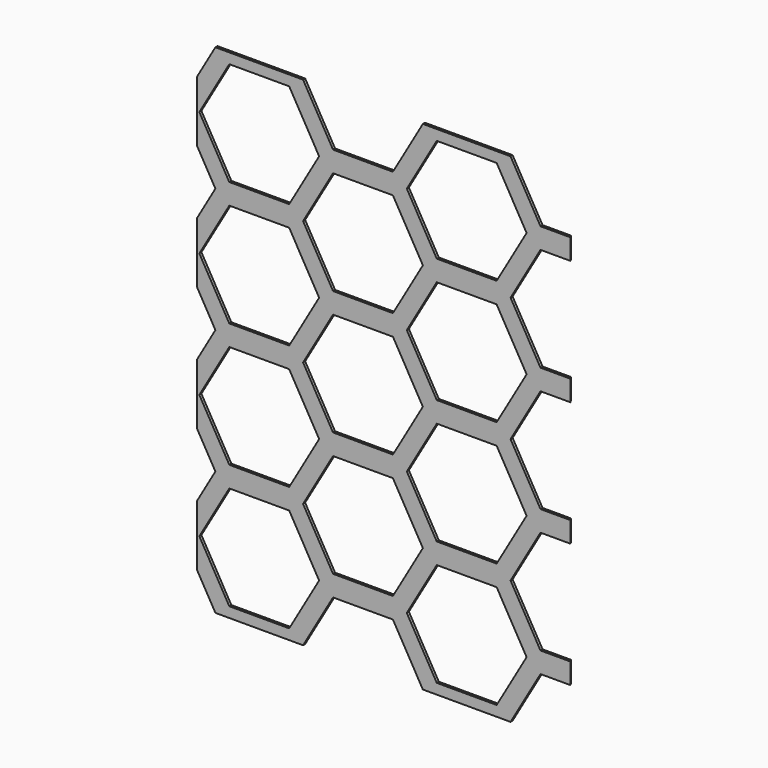
from build123d import *

# Parameters (mm, degrees)
F1_DEPTH    = 3.175
F2_T1_DEPTH = 41.9033921872
F3_T1_DEPTH = 42.5180012054
F4_T1_DEPTH = 41.9033921872
F5_T1_DEPTH = 41.9033921872


# Not quite as in the source:
# - a fillet or chamfer that OpenCascade refuses, or shapes differently, is made with other operations: its cross-section is extruded or revolved along the edge and cut away or added
# - ends of sketch curves that miss each other by under 0.0002 mm in the source are joined


with BuildPart() as f1:
    # F0 (on Front) → F1 (new body)
    with BuildSketch(Plane.XZ):
        Polygon((-134.9552678654, 118.4551059571), (-242.3083075974, 118.4551059571), (-264.8317917845, 79.4432945156), (-264.8317917845, 5.0669305831), (-242.3083075974, -33.9448883924), (-264.8317917845, -72.9567073679), (-264.8317917845, -147.3330713004), (-242.3083075974, -186.3448902759), (-264.8317917845, -225.3567092514), (-264.8317917845, -299.7330731839), (-242.3083075974, -338.7448921594), (-264.8317917845, -377.7567111349), (-264.8317917845, -452.1330750674), (-242.3083075974, -491.1448940429), (-134.9552678654, -491.1448940429), (-98.2935257718, -427.6448940429), (-24.9700415847, -427.6448940429), (11.6917005088, -491.1448940429), (119.0447402409, -491.1448940429), (155.7064823344, -427.6448940429), (192.3682082155, -427.6448940429), (192.3682082155, -402.2448921594), (155.7064823344, -402.2448921594), (119.0447402409, -338.7448921594), (155.7064823344, -275.2448921594), (192.3682082155, -275.2448921594), (192.3682082155, -249.8448902759), (155.7064823344, -249.8448902759), (119.0447402409, -186.3448902759), (155.7064823344, -122.8448902759), (192.3682082155, -122.8448902759), (192.3682082155, -97.4448883924), (155.7064823344, -97.4448883924), (119.0447402409, -33.9448883924), (155.7064823344, 29.5551116076), (192.3682082155, 29.5551116076), (192.3682082155, 54.9551134911), (155.7064823344, 54.9551134911), (119.0447402409, 118.4551134911), (11.6917005088, 118.4551059571), (-24.9700415847, 54.9551134911), (-98.2935257718, 54.9551134911), align=None)
        Polygon((-261.9552759716, -414.9448940429), (-225.2935338781, -351.4448940429), (-151.970049691, -351.4448940429), (-115.3083075974, -414.9448940429), (-151.970049691, -478.4448940429), (-225.2935338781, -478.4448940429), align=None, mode=Mode.SUBTRACT)
        Polygon((11.6917005088, -338.7448921594), (-24.9700415847, -402.2448921594), (-98.2935257718, -402.2448921594), (-134.9552678654, -338.7448921594), (-98.2935257718, -275.2448921594), (-24.9700415847, -275.2448921594), align=None, mode=Mode.SUBTRACT)
        Polygon((-115.3083075974, -262.5448921594), (-151.970049691, -326.0448921594), (-225.2935338781, -326.0448921594), (-261.9552759716, -262.5448921594), (-225.2935338781, -199.0448921594), (-151.970049691, -199.0448921594), align=None, mode=Mode.SUBTRACT)
        Polygon((138.6917005088, -414.9448940429), (102.0299584153, -478.4448940429), (28.7064742282, -478.4448940429), (-7.9552678654, -414.9448940429), (28.7064742282, -351.4448940429), (102.0299584153, -351.4448940429), align=None, mode=Mode.SUBTRACT)
        Polygon((138.6917005088, -262.5448921594), (102.0299584153, -326.0448921594), (28.7064742282, -326.0448921594), (-7.9552678654, -262.5448921594), (28.7064742282, -199.0448921594), (102.0299584153, -199.0448921594), align=None, mode=Mode.SUBTRACT)
        Polygon((-115.3083075974, -110.1448902759), (-151.970049691, -173.6448902759), (-225.2935338781, -173.6448902759), (-261.9552759716, -110.1448902759), (-225.2935338781, -46.6448902759), (-151.970049691, -46.6448902759), align=None, mode=Mode.SUBTRACT)
        Polygon((11.6917005088, -186.3448902759), (-24.9700415847, -249.8448902759), (-98.2935257718, -249.8448902759), (-134.9552678654, -186.3448902759), (-98.2935257718, -122.8448902759), (-24.9700415847, -122.8448902759), align=None, mode=Mode.SUBTRACT)
        Polygon((11.6917005088, -33.9448883924), (-24.9700415847, -97.4448883924), (-98.2935257718, -97.4448883924), (-134.9552678654, -33.9448883924), (-98.2935257718, 29.5551116076), (-24.9700415847, 29.5551116076), align=None, mode=Mode.SUBTRACT)
        Polygon((-115.3083075974, 42.2551116076), (-151.970049691, -21.2448883924), (-225.2935338781, -21.2448883924), (-261.9552759716, 42.2551116076), (-225.2935338781, 105.7551116076), (-151.970049691, 105.7551116076), align=None, mode=Mode.SUBTRACT)
        Polygon((138.6917005088, -110.1448902759), (102.0299584153, -173.6448902759), (28.7064742282, -173.6448902759), (-7.9552678654, -110.1448902759), (28.7064742282, -46.6448902759), (102.0299584153, -46.6448902759), align=None, mode=Mode.SUBTRACT)
        Polygon((138.6917005088, 42.2551116076), (102.0299584153, -21.2448883924), (28.7064742282, -21.2448883924), (-7.9552678654, 42.2551116076), (28.7064742282, 105.7551116076), (102.0299584153, 105.7551116076), align=None, mode=Mode.SUBTRACT)
    extrude(amount=F1_DEPTH)

    # F2: chamfer of 1.8415 x 3.1895715621 on 1 edges, made by hand

    # F2_s2 → F2_t1 (cut)
    with BuildSketch(Plane.XY.offset(21.3034164558)):
        Polygon((192.3682082155, -3.1895715621), (190.5267082155, 0), (192.3682082155, 0), align=None)
    extrude(amount=F2_T1_DEPTH, mode=Mode.SUBTRACT)

    # F3: chamfer of 1.91008 x 3.3083556065 on 1 edges, made by hand

    # F3_s2 → F3_t1 (cut)
    with BuildSketch(Plane.XY.offset(-131.4038899368)):
        Polygon((190.4581282155, 0), (192.3682082155, -3.3083556065), (192.3682082155, 0), align=None)
    extrude(amount=F3_T1_DEPTH, mode=Mode.SUBTRACT)

    # F4: chamfer of 1.8415 x 3.1895715621 on 1 edges, made by hand

    # F4_s2 → F4_t1 (cut)
    with BuildSketch(Plane.XY.offset(-283.4965873112)):
        Polygon((190.5267082155, 0), (192.3682082155, -3.1895715621), (192.3682082155, 0), align=None)
    extrude(amount=F4_T1_DEPTH, mode=Mode.SUBTRACT)

    # F5: chamfer of 1.8415 x 3.1895715621 on 1 edges, made by hand

    # F5_s2 → F5_t1 (cut)
    with BuildSketch(Plane.XY.offset(-435.8965891948)):
        Polygon((190.5267082155, 0), (192.3682082155, -3.1895715621), (192.3682082155, 0), align=None)
    extrude(amount=F5_T1_DEPTH, mode=Mode.SUBTRACT)


solid = f1.part
